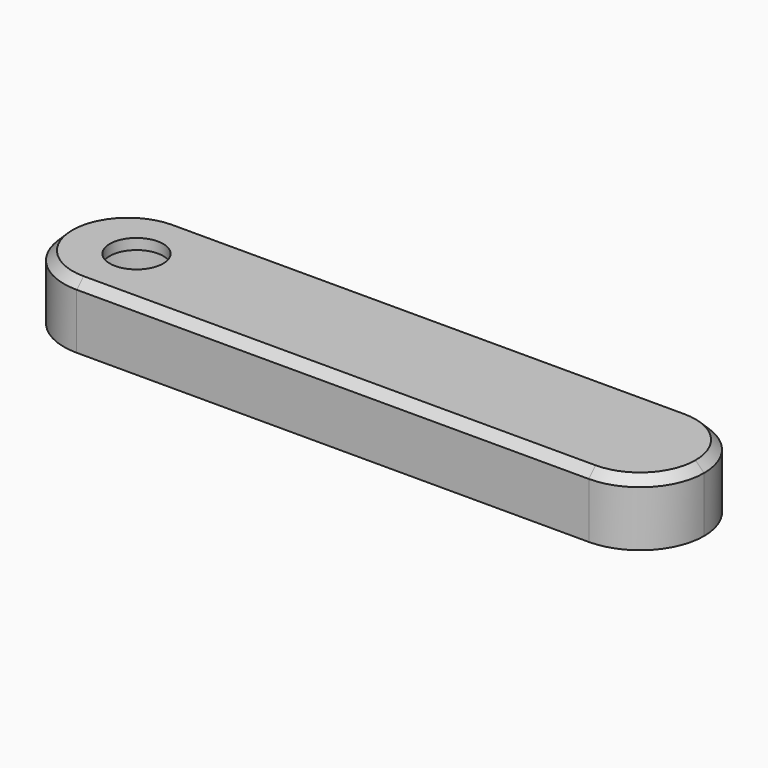
from build123d import *

# Parameters (mm, degrees)
F0_W     = 30
F0_H     = 6
F1_DEPTH = 3
F2_R     = 2.4
F2_R_2   = 1.25
F3_DEPTH = 2.5
F4_DEPTH = 3.001
F5_R     = 2.99999
F6_SIZE  = 0.4


# Not quite as in the source:
# - a fillet or chamfer is up to 0.001 mm smaller than in the source, because OpenCascade refuses the exact size


with BuildPart() as f1:
    # F0 (on Top) → F1 (new body)
    with BuildSketch(Plane.XY):
        with Locations((15, 0)):
            Rectangle(F0_W, F0_H)
    extrude(amount=F1_DEPTH)

    # F2 (on face) → F3 (cut)
    with BuildSketch(Plane(origin=(0, 0, 0), x_dir=(1, 0, 0), z_dir=(0, 0, -1))):
        with Locations((3.4, 0)):
            Circle(F2_R)
        with Locations((3.4, 0)):
            Circle(F2_R_2, mode=Mode.SUBTRACT)
        with Locations((3.4, 0)):
            Circle(F2_R_2)
    extrude(amount=-F3_DEPTH, mode=Mode.SUBTRACT)

    # F2 (on face) → F4 (cut, through all)
    with BuildSketch(Plane(origin=(0, 0, 0), x_dir=(1, 0, 0), z_dir=(0, 0, -1))):
        with Locations((3.4, 0)):
            Circle(F2_R_2)
    extrude(amount=-F4_DEPTH, mode=Mode.SUBTRACT)

    # F5 (radius 3 in the source; OpenCascade refuses exactly that, so slightly less here)
    f5_edges = [f1.edges().sort_by_distance(p)[0] for p in [
        (0, -3, 1.5),
        (0, 3, 1.5),
        (30, -3, 1.5),
        (30, 3, 1.5),
    ]]
    fillet(f5_edges, radius=F5_R)

    # F6
    f6_edges = [f1.edges().sort_by_distance(p)[0] for p in [
        (15, 3, 3),
    ]]
    chamfer(f6_edges, length=F6_SIZE)


solid = f1.part
